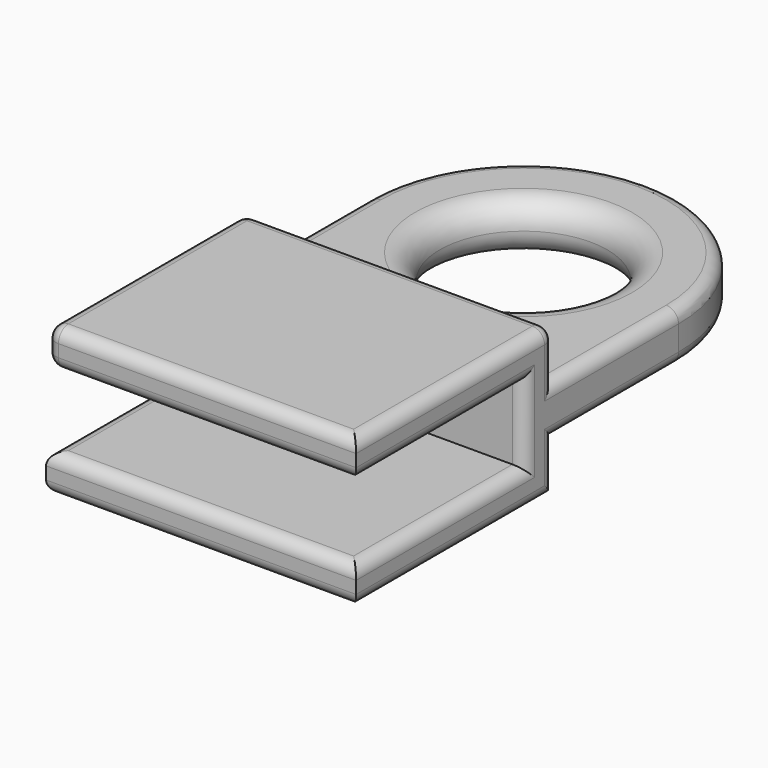
from build123d import *

# Parameters (mm, degrees)
F0_W     = 31.75
F0_H     = 25.4
F1_DEPTH = 3.81
F2_W     = 31.75
F2_H     = 3.81
F3_DEPTH = 3.81
F5_W     = 31.75
F5_H     = 5.08
F6_DEPTH = 31.75
F7_R     = 8.5850562929
F8_DEPTH = 10.161
F9_R     = 15.875
F10_R    = 15.87499
F11_R    = 1.27
F12_R    = 2.53999


# Not quite as in the source:
# - a fillet or chamfer is up to 0.001 mm smaller than in the source, because OpenCascade refuses the exact size


with BuildPart() as f1:
    # F0 (on Top) → F1 (new body)
    with BuildSketch(Plane.XY):
        with Locations((1.8298272586, 1.9303451554)):
            Rectangle(F0_W, F0_H)
    extrude(amount=F1_DEPTH)

    # F2 (on face) → F3 (join)
    with BuildSketch(Plane.XY.offset(3.81)):
        with Locations((1.8298272586, 12.7253451554)):
            Rectangle(F2_W, F2_H)
    extrude(amount=F3_DEPTH)

    # F4: F1 across face


with BuildPart() as f1_1:
    add(f1.part)
    add(f1.part.mirror(Plane(origin=(1.8298272586, 12.7253451554, 7.62), x_dir=(1, 0, 0), z_dir=(0, 0, 1))))

    # F5 (on face) → F6 (join)
    with BuildSketch(Plane(origin=(0, 14.6303451554, 0), x_dir=(-1, 0, 0), z_dir=(0, 1, 0))):
        with Locations((-1.8298272586, 7.62)):
            Rectangle(F5_W, F5_H)
    extrude(amount=F6_DEPTH)

    # F7 (on face) → F8 (cut, through all)
    with BuildSketch(Plane(origin=(0, 0, 5.08), x_dir=(1, 0, 0), z_dir=(0, 0, -1))):
        with Locations((1.8298272586, -30.5053451554)):
            Circle(F7_R)
    extrude(amount=-F8_DEPTH, mode=Mode.SUBTRACT)

    # F9
    f9_edges = [f1_1.edges().sort_by_distance(p)[0] for p in [
        (17.704827, 46.380345, 7.62),
    ]]
    fillet(f9_edges, radius=F9_R)

    # F10 (radius 15.875 in the source; OpenCascade refuses exactly that, so slightly less here)
    f10_edges = [f1_1.edges().sort_by_distance(p)[0] for p in [
        (-14.045173, 46.380345, 7.62),
    ]]
    fillet(f10_edges, radius=F10_R)

    # F11
    f11_edges = [f1_1.edges().sort_by_distance(p)[0] for p in [
        (-14.045173, -10.769655, 13.335),
        (-14.045173, 0.025345, 11.43),
        (-14.045173, 1.930345, 15.24),
        (-14.045173, 0.025345, 3.81),
        (-14.045173, 1.930345, 0),
        (-14.045173, 10.820345, 7.62),
        (-14.045173, 22.56785, 10.16),
        (-14.045173, 22.56785, 5.08),
        (1.829827, 14.630345, 15.24),
        (-14.045173, 14.630345, 12.7),
        (-14.045173, 14.630345, 2.54),
        (1.829827, -10.769655, 3.81),
        (1.829827, -10.769655, 11.43),
        (1.829827, -10.769655, 0),
        (1.829827, -10.769655, 15.24),
        (17.704827, 1.930345, 15.24),
        (17.704827, 0.025345, 11.43),
        (17.704827, 0.025345, 3.81),
        (17.704827, 1.930345, 0),
        (17.704827, 14.630345, 2.54),
        (17.704827, 14.630345, 12.7),
        (17.704827, 10.820345, 7.62),
    ]]
    fillet(f11_edges, radius=F11_R)

    # F12 (radius 2.54 in the source; OpenCascade refuses exactly that, so slightly less here)
    f12_edges = [f1_1.edges().sort_by_distance(p)[0] for p in [
        (-6.755229, 30.505345, 10.16),
        (-6.755229, 30.505345, 5.08),
    ]]
    fillet(f12_edges, radius=F12_R)


solid = f1_1.part
